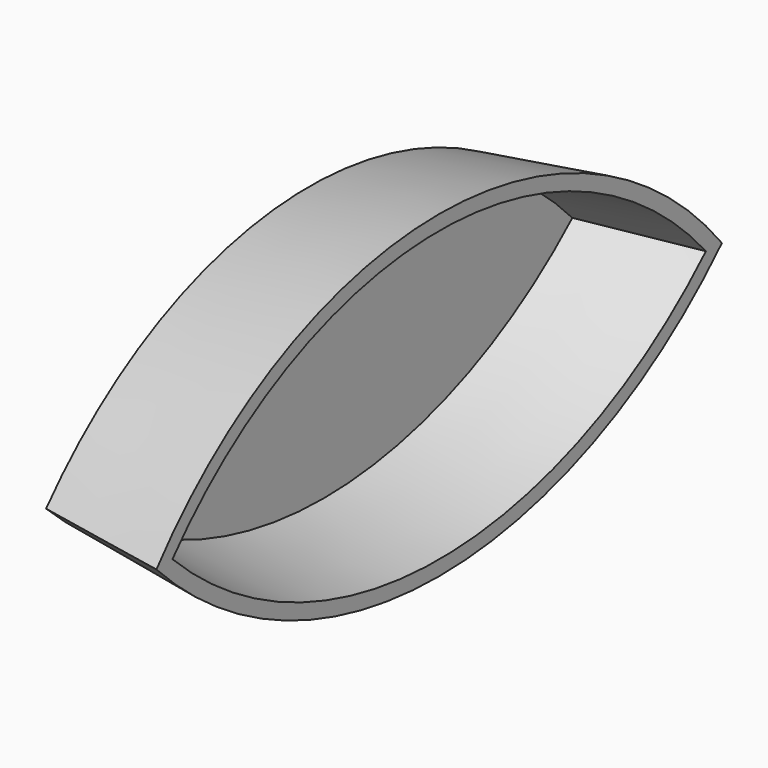
from build123d import *

# Parameters (mm, degrees)
F1_DEPTH               = 26.6
DRAFT_F1_DRAFTED_ANGLE = -8
F2_T                   = 3


# Not quite as in the source:
# - an extrude with a draft is written as a straight extrude whose walls are then drafted
# - a shell that OpenCascade refuses in one call is made with other operations: the cavity is built on its own and cut out


with BuildPart() as f1:
    # F0 (on Right) → F1 (new body)
    with BuildSketch(Plane.YZ):
        with BuildLine():
            ThreePointArc((-67.9076090455, 0), (-0.7408112288, -27.0852345678), (66.425986588, 0))
            ThreePointArc((66.425986588, 0), (-0.7408112288, 30.6287280565), (-67.9076090455, 0))
        make_face()
    extrude(amount=F1_DEPTH)

    # draft_F1_drafted
    draft_f1_drafted_walls = [f1.faces().sort_by_distance(p)[0] for p in [
        (17.7333333333, -0.7408112288, -27.0852345678),
        (17.7333333333, -0.7408112288, 30.6287280565),
    ]]
    draft(draft_f1_drafted_walls, neutral_plane=Plane.YZ, angle=DRAFT_F1_DRAFTED_ANGLE)

    # F2: shell of thickness 3, made by hand


with BuildPart() as f2_core1:
    # F2_t2: copy of F1
    add(f1.part)

    # the walls: a layer under each face that stays
    f2_faces = [f2_core1.faces().sort_by_distance(p)[0] for p in [
        (13.3, -0.7408112288, -28.9544276693),
        (13.3, -0.7408112288, 32.4979211581),
        (0, -0.7408112288, 1.7717467444),
    ]]
    thicken(f2_faces, amount=-F2_T, mode=Mode.SUBTRACT)


with BuildPart() as f1_1:
    add(f1.part)

    # what is left inside the walls is the cavity
    f2_cavity = [f2_core1.part.solids().sort_by_distance(p)[0] for p in [
        (26.57, -0.740811, -8.083548),
    ]]
    add(f2_cavity, mode=Mode.SUBTRACT)


solid = f1_1.part
